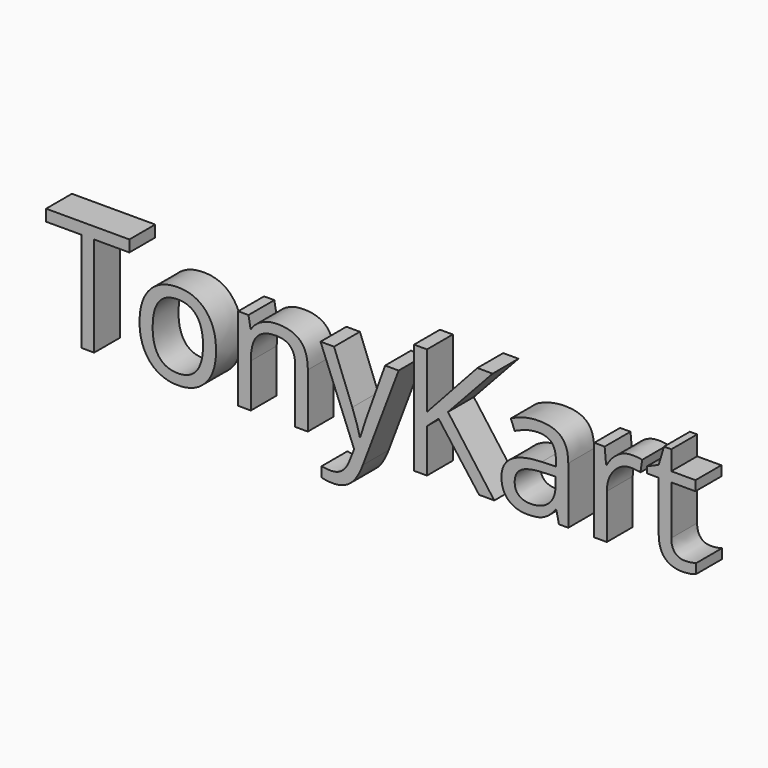
from build123d import *

# Parameters (mm, degrees)
F0_TEXT_SIZE = 122.3579618252
F1_DEPTH     = 25.4


# Not quite as in the source:
# - Text() gives the source's letters only with a copy of the font that has no kerning and outlines rounded to 1/6400 em; it was checked with that copy


with BuildPart() as f1:
    # F0 (on Front) → F1 (new body)
    with BuildSketch(Plane.XZ):
        with Locations((-438.9596655965, -38.7385338545)):
            Text('TonyKart', F0_TEXT_SIZE, font='Open Sans', text_align=(TextAlign.LEFT, TextAlign.BOTTOM))
    extrude(amount=F1_DEPTH)


solid = f1.part
